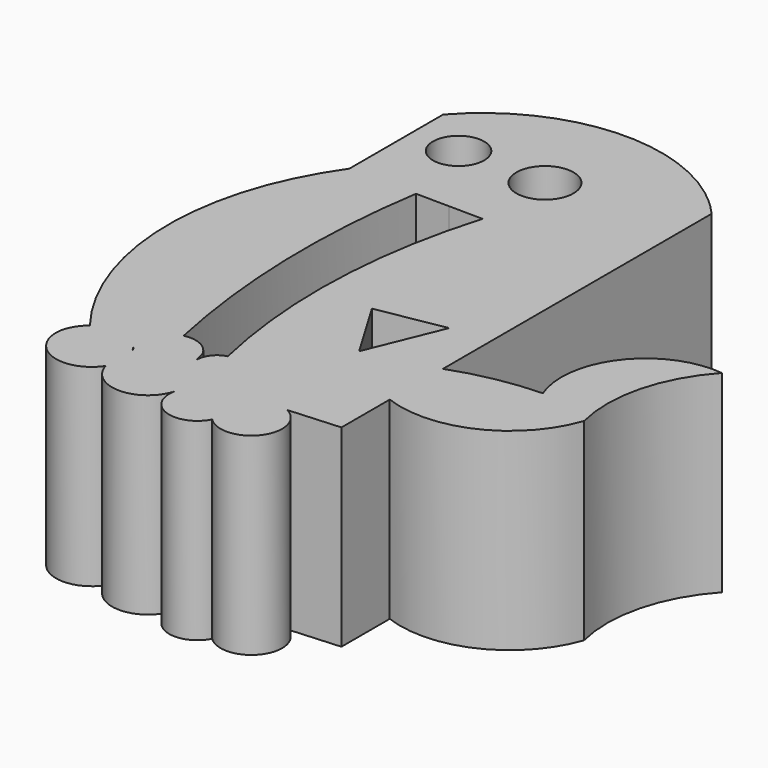
from build123d import *

# Parameters (mm, degrees)
F0_R     = 3.3686848121
F0_R_2   = 3.7503411647
F1_DEPTH = 25.4


# Not quite as in the source:
# - the program builds the solid bodies; features that only make, move or delete a surface that nothing else refers to are left out


with BuildPart() as f1:
    # F0 (on Top) → F1 (new body)
    with BuildSketch(Plane.XY):
        with BuildLine():
            Line((-11.4056267505, -5.9082075022), (-11.4056267505, 38.28210113))
            ThreePointArc((-11.4056267505, 38.28210113), (-13.0902542949, 40.0050046024), (-14.9420781413, 41.5467940758))
            ThreePointArc((-14.9420781413, 41.5467940758), (-24.4960295494, 45.8046369765), (-34.9515650706, 45.5063239844))
            ThreePointArc((-34.9515650706, 45.5063239844), (-41.3833712338, 42.777482568), (-46.7318524877, 38.28210113))
            Line((-46.7318524877, 38.28210113), (-46.7318524877, 22.8735643321))
            Line((-46.7318524877, 22.8735643321), (-37.9002960534, 22.7850040211))
            Line((-37.9002960534, 22.7850040211), (-33.5099794506, 22.7409791874))
            Line((-33.5099794506, 22.7409791874), (-29.0687396191, 22.6964437101))
            ThreePointArc((-29.0687396191, 22.6964437101), (-32.3476402886, 2.6663309949), (-30.4037962217, -17.5370864196))
            ThreePointArc((-30.4037962217, -17.5370864196), (-28.3292963567, -17.9171307498), (-27.2098111607, -19.7045132715))
            ThreePointArc((-27.2098111607, -19.7045132715), (-22.8158840867, -19.1811881286), (-19.9977839656, -22.5927531719))
            ThreePointArc((-19.9977839656, -22.5927531719), (-19.0499304153, -22.7087900697), (-18.1556105797, -23.043577982))
            Line((-18.1556105797, -23.043577982), (-11.4056267505, -22.5927531719))
            Line((-11.4056267505, -22.5927531719), (-11.4056267505, -14.6515189691))
            ThreePointArc((-11.4056267505, -14.6515189691), (-0.2868217682, -14.1752443759), (7.1637327783, -5.9082075022))
            ThreePointArc((7.1637327783, -5.9082075022), (7.197230267, 3.2378107083), (11.5452415215, 11.2842738641))
            ThreePointArc((11.5452415215, 11.2842738641), (1.5408183988, 7.0311325334), (0, -3.7300742697))
            ThreePointArc((0, -3.7300742697), (-5.7908190197, -4.3583061138), (-11.4056267505, -5.9082075022))
        make_face()
        Polygon((-25.470810011, 0), (-16.5671050976, 1.5869429488), (-20.5766428262, -8.2222158089), align=None, mode=Mode.SUBTRACT)
        with Locations((-40.4367111623, 32.953761518)):
            Circle(F0_R, mode=Mode.SUBTRACT)
        with Locations((-29.0687396191, 32.953761518)):
            Circle(F0_R_2, mode=Mode.SUBTRACT)
        with BuildLine():
            Line((-37.9002960534, 22.7850040211), (-46.7318524877, 22.8735643321))
            ThreePointArc((-46.7318524877, 22.8735643321), (-53.4771270799, 0.7607999274), (-45.7492200512, -21.028016743))
            ThreePointArc((-45.7492200512, -21.028016743), (-44.0238078591, -20.1849073614), (-42.104174186, -20.131174475))
            ThreePointArc((-42.104174186, -20.131174475), (-40.558011078, -20.7291440142), (-39.3299119733, -21.8426791577))
            ThreePointArc((-39.3299119733, -21.8426791577), (-39.2808229847, -18.7066363859), (-36.8050348739, -16.7811112041))
            ThreePointArc((-36.8050348739, -16.7811112041), (-39.1633371869, 2.951823761), (-37.9002960534, 22.7850040211))
        make_face()
        with BuildLine():
            ThreePointArc((-42.104174186, -20.131174475), (-44.0238078591, -20.1849073614), (-45.7492200512, -21.028016743))
            ThreePointArc((-45.7492200512, -21.028016743), (-46.9337681485, -22.4383900317), (-47.4600126918, -24.2034321528))
            ThreePointArc((-47.4600126918, -24.2034321528), (-44.2480891567, -28.8954606668), (-38.8667027357, -27.059088003))
            ThreePointArc((-38.8667027357, -27.059088003), (-34.3322542596, -30.4586049869), (-29.7978057834, -27.059088003))
            ThreePointArc((-29.7978057834, -27.059088003), (-27.4071947516, -31.3060964302), (-22.8805579245, -29.5000895858))
            ThreePointArc((-22.8805579245, -29.5000895858), (-16.7448352708, -29.0331395554), (-18.1556105797, -23.043577982))
            ThreePointArc((-18.1556105797, -23.043577982), (-19.0499304153, -22.7087900697), (-19.9977839656, -22.5927531719))
            ThreePointArc((-19.9977839656, -22.5927531719), (-22.8158840867, -19.1811881286), (-27.2098111607, -19.7045132715))
            ThreePointArc((-27.2098111607, -19.7045132715), (-28.3292963567, -17.9171307498), (-30.4037962217, -17.5370864196))
            ThreePointArc((-30.4037962217, -17.5370864196), (-31.8655744774, -18.4799458919), (-32.4125880239, -20.131174475))
            ThreePointArc((-32.4125880239, -20.131174475), (-32.5829263413, -19.4613489943), (-32.7484000877, -18.7903052132))
            ThreePointArc((-32.7484000877, -18.7903052132), (-34.4248384474, -17.0752518162), (-36.8050348739, -16.7811112041))
            ThreePointArc((-36.8050348739, -16.7811112041), (-39.2808229847, -18.7066363859), (-39.3299119733, -21.8426791577))
            ThreePointArc((-39.3299119733, -21.8426791577), (-40.558011078, -20.7291440142), (-42.104174186, -20.131174475))
        make_face()
        with BuildLine():
            ThreePointArc((-38.8667027357, -22.5927531719), (-39.1211782585, -22.231840123), (-39.3299119733, -21.8426791577))
            ThreePointArc((-39.3299119733, -21.8426791577), (-39.0800443488, -22.2064378205), (-38.8667027357, -22.5927531719))
        make_face(mode=Mode.SUBTRACT)
    extrude(amount=F1_DEPTH)


solid = f1.part
